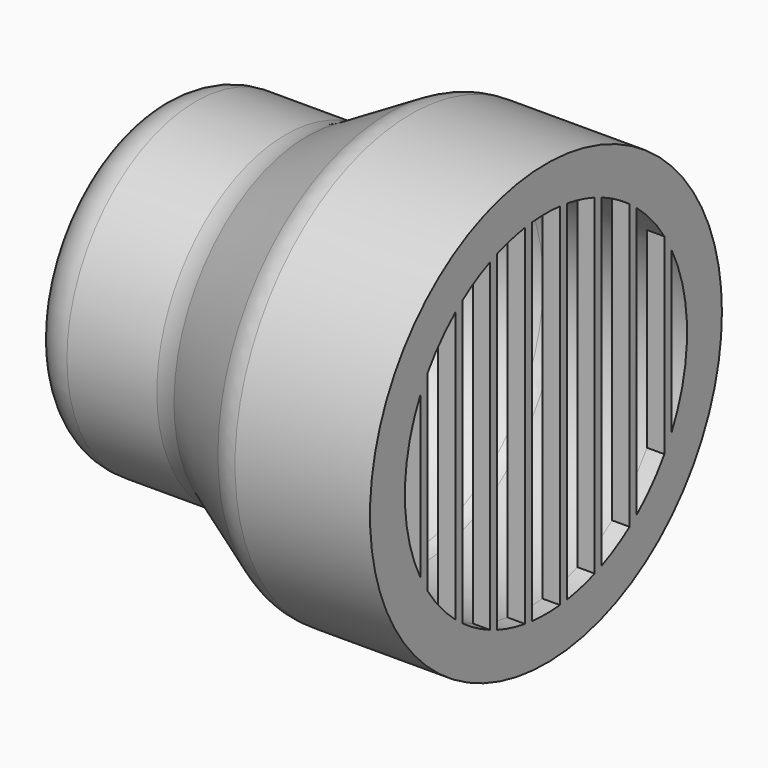
from build123d import *

# Parameters (mm, degrees)
F2_R     = 25.25
F3_DEPTH = 2
F5_DEPTH = 2
F6_R     = 4.99999
F7_R     = 3


# Not quite as in the source:
# - a fillet or chamfer is up to 0.001 mm smaller than in the source, because OpenCascade refuses the exact size
# - a feature names something its author has since deleted; it is built from what else it names


with BuildPart() as f1:
    # F0 (on Top) → F1 (revolve)
    with BuildSketch(Plane.XY):
        Polygon((-18, 18.5), (-18, 13.5), (0, 13.5), (11.6913429511, 20.25), (25.1913429511, 20.25), (25.1913429511, 25.25), (10.3515969889, 25.25), (-1.3397459622, 18.5), align=None)
    revolve(axis=Axis((-8.7595172226, 0, 0), (1, 0, 0)))

    # F2 (on face) → F3 (join)
    with BuildSketch(Plane.YZ.offset(25.1913429511)):
        Circle(F2_R)
    extrude(amount=F3_DEPTH)

    # F4 (on face) → F5 (cut, through all)
    with BuildSketch(Plane.YZ.offset(27.1913429511)):
        with BuildLine():
            ThreePointArc((17, 11.0028405423), (15.1695473581, 13.4144449363), (13, 15.5261875552))
            Line((13, 15.5261875552), (13, -15.5261875552))
            ThreePointArc((13, -15.5261875552), (15.1695473581, -13.4144449363), (17, -11.0028405423))
            Line((17, -11.0028405423), (17, 11.0028405423))
        make_face()
        with BuildLine():
            ThreePointArc((12, 16.3114223782), (10.0654136275, 17.5712819255), (8, 18.6027551723))
            Line((8, 18.6027551723), (8, -18.6027551723))
            ThreePointArc((8, -18.6027551723), (10.0654136275, -17.5712819255), (12, -16.3114223782))
            Line((12, -16.3114223782), (12, 16.3114223782))
        make_face()
        with BuildLine():
            ThreePointArc((7, 19.0016446657), (5.0261919098, 19.6163170571), (3, 20.0265448842))
            Line((3, 20.0265448842), (3, -20.0265448842))
            ThreePointArc((3, -20.0265448842), (5.0261919098, -19.6163170571), (7, -19.0016446657))
            Line((7, -19.0016446657), (7, 19.0016446657))
        make_face()
        with BuildLine():
            ThreePointArc((2, 20.1509925314), (0, 20.25), (-2, 20.1509925314))
            Line((-2, 20.1509925314), (-2, -20.1509925314))
            ThreePointArc((-2, -20.1509925314), (0, -20.25), (2, -20.1509925314))
            Line((2, -20.1509925314), (2, 20.1509925314))
        make_face()
        with BuildLine():
            Line((-3, -20.0265448842), (-3, 20.0265448842))
            ThreePointArc((-3, 20.0265448842), (-5.0261919098, 19.6163170571), (-7, 19.0016446657))
            Line((-7, 19.0016446657), (-7, -19.0016446657))
            ThreePointArc((-7, -19.0016446657), (-5.0261919098, -19.6163170571), (-3, -20.0265448842))
        make_face()
        with BuildLine():
            Line((-8, -18.6027551723), (-8, 18.6027551723))
            ThreePointArc((-8, 18.6027551723), (-10.0654136275, 17.5712819255), (-12, 16.3114223782))
            Line((-12, 16.3114223782), (-12, -16.3114223782))
            ThreePointArc((-12, -16.3114223782), (-10.0654136275, -17.5712819255), (-8, -18.6027551723))
        make_face()
        with BuildLine():
            Line((-13, -15.5261875552), (-13, 15.5261875552))
            ThreePointArc((-13, 15.5261875552), (-15.1695473581, 13.4144449363), (-17, 11.0028405423))
            Line((-17, 11.0028405423), (-17, -11.0028405423))
            ThreePointArc((-17, -11.0028405423), (-15.1695473581, -13.4144449363), (-13, -15.5261875552))
        make_face()
        with BuildLine():
            Line((-18, -9.2769876576), (-18, 9.2769876576))
            ThreePointArc((-18, 9.2769876576), (-20.25, 0), (-18, -9.2769876576))
        make_face()
        with BuildLine():
            ThreePointArc((20.25, 0), (19.6794626451, 4.772970773), (18, 9.2769876576))
            Line((18, 9.2769876576), (18, -9.2769876576))
            ThreePointArc((18, -9.2769876576), (19.6794626451, -4.772970773), (20.25, 0))
        make_face()
    extrude(amount=-F5_DEPTH, mode=Mode.SUBTRACT)

    # F6 (radius 5 in the source; OpenCascade refuses exactly that, so slightly less here)
    f6_edges = [f1.edges().sort_by_distance(p)[0] for p in [
        (-18, -18.5, 0),
        (-1.339746, -18.5, 0),
        (10.351597, -25.25, 0),
    ]]
    fillet(f6_edges, radius=F6_R)

    # F7
    f7_edges = [f1.edges().sort_by_distance(p)[0] for p in [
        (11.691343, -20.25, 0),
        (0, -13.5, 0),
    ]]
    fillet(f7_edges, radius=F7_R)


solid = f1.part
